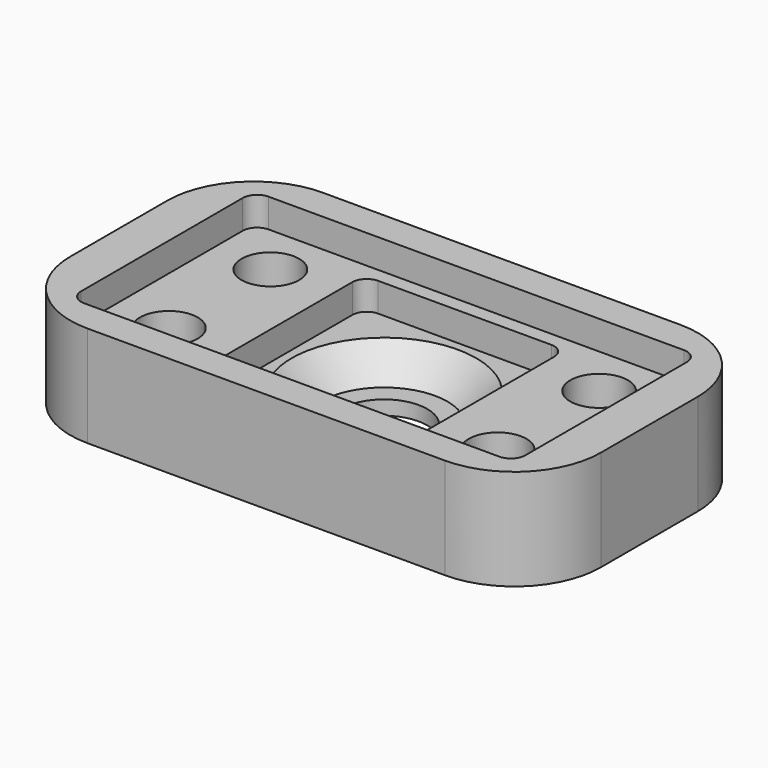
from build123d import *

# Parameters (mm, degrees)
F0_R     = 1
F0_R_2   = 1.5
F1_DEPTH = 0.5
F2_R     = 1
F2_R_2   = 2.2
F3_DEPTH = 1
F4_SIZE  = 0.99999
F5_R     = 1
F6_DEPTH = 1
F8_DEPTH = 1


# Not quite as in the source:
# - a fillet or chamfer is up to 0.001 mm smaller than in the source, because OpenCascade refuses the exact size


with BuildPart() as f1:
    # F0 (on Top) → F1 (new body)
    with BuildSketch(Plane.XY):
        with BuildLine():
            Line((-6.2, -5.1), (6.2, -5.1))
            ThreePointArc((6.2, -5.1), (8.3213203436, -4.2213203436), (9.2, -2.1))
            Line((9.2, -2.1), (9.2, 2.1))
            ThreePointArc((9.2, 2.1), (8.3213203436, 4.2213203436), (6.2, 5.1))
            Line((6.2, 5.1), (-6.2, 5.1))
            ThreePointArc((-6.2, 5.1), (-8.3213203436, 4.2213203436), (-9.2, 2.1))
            Line((-9.2, 2.1), (-9.2, -2.1))
            ThreePointArc((-9.2, -2.1), (-8.3213203436, -4.2213203436), (-6.2, -5.1))
        make_face()
        with Locations((-5.7, -2.2)):
            Circle(F0_R, mode=Mode.SUBTRACT)
        with Locations((5.7, -2.2)):
            Circle(F0_R, mode=Mode.SUBTRACT)
        with Locations((-5.7, 2.2)):
            Circle(F0_R, mode=Mode.SUBTRACT)
        Circle(F0_R_2, mode=Mode.SUBTRACT)
        with Locations((5.7, 2.2)):
            Circle(F0_R, mode=Mode.SUBTRACT)
    extrude(amount=F1_DEPTH)

    # F2 (on face) → F3 (join)
    with BuildSketch(Plane.XY.offset(0.5)):
        with BuildLine():
            ThreePointArc((-6.2, 5.1), (-8.3213203436, 4.2213203436), (-9.2, 2.1))
            Line((-9.2, 2.1), (-9.2, -2.1))
            ThreePointArc((-9.2, -2.1), (-8.3213203436, -4.2213203436), (-6.2, -5.1))
            Line((-6.2, -5.1), (6.2, -5.1))
            ThreePointArc((6.2, -5.1), (8.3213203436, -4.2213203436), (9.2, -2.1))
            Line((9.2, -2.1), (9.2, 2.1))
            ThreePointArc((9.2, 2.1), (8.3213203436, 4.2213203436), (6.2, 5.1))
            Line((6.2, 5.1), (-6.2, 5.1))
        make_face()
        with Locations((-5.7, -2.2)):
            Circle(F2_R, mode=Mode.SUBTRACT)
        Circle(F2_R_2, mode=Mode.SUBTRACT)
        with Locations((5.7, -2.2)):
            Circle(F2_R, mode=Mode.SUBTRACT)
        with Locations((-5.7, 2.2)):
            Circle(F2_R, mode=Mode.SUBTRACT)
        with Locations((5.7, 2.2)):
            Circle(F2_R, mode=Mode.SUBTRACT)
    extrude(amount=F3_DEPTH)

    # F4 (size 1 in the source; OpenCascade refuses exactly that, so slightly less here)
    f4_edges = [f1.edges().sort_by_distance(p)[0] for p in [
        (-2.2, 0, 1.5),
    ]]
    chamfer(f4_edges, length=F4_SIZE)

    # F5 (on face) → F6 (join)
    with BuildSketch(Plane.XY.offset(1.5)):
        with BuildLine():
            Line((6.2, 5.1), (-6.2, 5.1))
            ThreePointArc((-6.2, 5.1), (-8.3213203436, 4.2213203436), (-9.2, 2.1))
            Line((-9.2, 2.1), (-9.2, -2.1))
            ThreePointArc((-9.2, -2.1), (-8.3213203436, -4.2213203436), (-6.2, -5.1))
            Line((-6.2, -5.1), (6.2, -5.1))
            ThreePointArc((6.2, -5.1), (8.3213203436, -4.2213203436), (9.2, -2.1))
            Line((9.2, -2.1), (9.2, 2.1))
            ThreePointArc((9.2, 2.1), (8.3213203436, 4.2213203436), (6.2, 5.1))
        make_face()
        with Locations((-5.7, -2.2)):
            Circle(F5_R, mode=Mode.SUBTRACT)
        with BuildLine():
            ThreePointArc((3.5, -3), (3.3535533906, -3.3535533906), (3, -3.5))
            Line((3, -3.5), (-3, -3.5))
            ThreePointArc((-3, -3.5), (-3.3535533906, -3.3535533906), (-3.5, -3))
            Line((-3.5, -3), (-3.5, 3))
            ThreePointArc((-3.5, 3), (-3.3535533906, 3.3535533906), (-3, 3.5))
            Line((-3, 3.5), (3, 3.5))
            ThreePointArc((3, 3.5), (3.3535533906, 3.3535533906), (3.5, 3))
            Line((3.5, 3), (3.5, -3))
        make_face(mode=Mode.SUBTRACT)
        with Locations((5.7, -2.2)):
            Circle(F5_R, mode=Mode.SUBTRACT)
        with Locations((-5.7, 2.2)):
            Circle(F5_R, mode=Mode.SUBTRACT)
        with Locations((5.7, 2.2)):
            Circle(F5_R, mode=Mode.SUBTRACT)
    extrude(amount=F6_DEPTH)

    # F7 (on face) → F8 (join)
    with BuildSketch(Plane.XY.offset(2.5)):
        with BuildLine():
            ThreePointArc((6.2, -5.1), (8.3213203436, -4.2213203436), (9.2, -2.1))
            Line((9.2, -2.1), (9.2, 2.1))
            ThreePointArc((9.2, 2.1), (8.3213203436, 4.2213203436), (6.2, 5.1))
            Line((6.2, 5.1), (-6.2, 5.1))
            ThreePointArc((-6.2, 5.1), (-8.3213203436, 4.2213203436), (-9.2, 2.1))
            Line((-9.2, 2.1), (-9.2, -2.1))
            ThreePointArc((-9.2, -2.1), (-8.3213203436, -4.2213203436), (-6.2, -5.1))
            Line((-6.2, -5.1), (6.2, -5.1))
        make_face()
        with BuildLine():
            ThreePointArc((7.7, -3.5), (7.5535533906, -3.8535533906), (7.2, -4))
            Line((7.2, -4), (-7.2, -4))
            ThreePointArc((-7.2, -4), (-7.5535533906, -3.8535533906), (-7.7, -3.5))
            Line((-7.7, -3.5), (-7.7, 3.5))
            ThreePointArc((-7.7, 3.5), (-7.5535533906, 3.8535533906), (-7.2, 4))
            Line((-7.2, 4), (7.2, 4))
            ThreePointArc((7.2, 4), (7.5535533906, 3.8535533906), (7.7, 3.5))
            Line((7.7, 3.5), (7.7, -3.5))
        make_face(mode=Mode.SUBTRACT)
    extrude(amount=F8_DEPTH)


solid = f1.part
